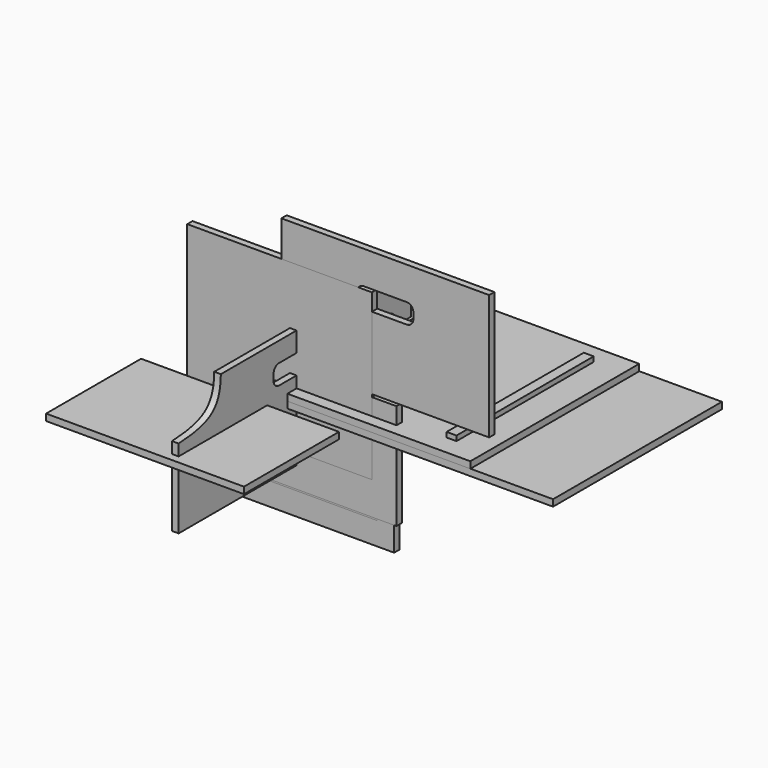
from build123d import *

# Parameters (mm, degrees)
F0_W      = 558.8
F0_H      = 406.4
F0_W_2    = 457.2
F0_H_2    = 19.05
F0_W_3    = 19.05
F0_H_3    = 241.3
F1_DEPTH  = 12.7
F2_DEPTH  = 22.225
F3_DEPTH  = 22.225
F4_DEPTH  = 22.225
F5_W      = 457.2
F5_H      = 406.4
F5_W_2    = 19.05
F5_H_2    = 330.2
F6_DEPTH  = 12.7
F7_DEPTH  = 22.225
F8_DEPTH  = 22.225
F9_W      = 406.4
F9_H      = 165.1
F10_DEPTH = 12.7
F12_DEPTH = 12.7
F13_W     = 381
F13_H     = 228.6
F14_DEPTH = 12.7
F15_W     = 400.05
F15_H     = 241.3
F16_DEPTH = 12.7
F17_W     = 317.5
F17_H     = 203.2
F18_DEPTH = 12.7
F19_W     = 381
F19_H     = 203.2
F20_DEPTH = 12.7
F21_W     = 355.6
F21_H     = 317.5
F22_DEPTH = 12.7


with BuildPart() as f1:
    # F0 (on Top) → F1 (new body)
    with BuildSketch(Plane.XY):
        with Locations((244.6383737266, 168.6325731099)):
            Rectangle(F0_W, F0_H)
        with Locations((206.5383737266, 0.3575731099)):
            Rectangle(F0_W_2, F0_H_2, mode=Mode.SUBTRACT)
        with Locations((206.5383737266, 336.9075731099)):
            Rectangle(F0_W_2, F0_H_2, mode=Mode.SUBTRACT)
        with Locations((489.1133737266, 168.6325731099)):
            Rectangle(F0_W_3, F0_H_3, mode=Mode.SUBTRACT)
    extrude(amount=-F1_DEPTH)

    # F0 (on Top) → F2 (join)
    with BuildSketch(Plane.XY):
        with Locations((206.5383737266, 336.9075731099)):
            Rectangle(F0_W_2, F0_H_2)
    extrude(amount=-F2_DEPTH)

    # F0 (on Top) → F3 (join)
    with BuildSketch(Plane.XY):
        with Locations((489.1133737266, 168.6325731099)):
            Rectangle(F0_W_3, F0_H_3)
    extrude(amount=-F3_DEPTH)

    # F0 (on Top) → F4 (join)
    with BuildSketch(Plane.XY):
        with Locations((206.5383737266, 0.3575731099)):
            Rectangle(F0_W_2, F0_H_2)
    extrude(amount=-F4_DEPTH)


with BuildPart() as f6:
    # F5 (on Top) → F6 (new body)
    with BuildSketch(Plane.XY):
        with Locations((136.398, 168.3692485094)):
            Rectangle(F5_W, F5_H)
        with Locations((9.525, 168.3692485094)):
            Rectangle(F5_W_2, F5_H_2, mode=Mode.SUBTRACT)
        with Locations((298.323, 168.3692485094)):
            Rectangle(F5_W_2, F5_H_2, mode=Mode.SUBTRACT)
    extrude(amount=F6_DEPTH)

    # F5 (on Top) → F7 (join)
    with BuildSketch(Plane.XY):
        with Locations((9.525, 168.3692485094)):
            Rectangle(F5_W_2, F5_H_2)
    extrude(amount=F7_DEPTH)

    # F5 (on Top) → F8 (join)
    with BuildSketch(Plane.XY):
        with Locations((298.323, 168.3692485094)):
            Rectangle(F5_W_2, F5_H_2)
    extrude(amount=F8_DEPTH)


with BuildPart() as f10:
    # F9 (on Front) → F10 (new body)
    with BuildSketch(Plane.XZ):
        with Locations((-2.5245882571, -122.1894112668)):
            Rectangle(F9_W, F9_H)
    extrude(amount=F10_DEPTH)


with BuildPart() as f12:
    # F11 (on Right) → F12 (new body)
    with BuildSketch(Plane.YZ):
        with BuildLine():
            Line((-106.0334625381, 110.8109265052), (-194.9334625381, 110.8109265052))
            add(Edge.make_bspline(
                [(-296.5334625381, 34.6109265052), (-215.7922492521, 38.1965605335), (-196.2180797117, 57.5377674894), (-194.9334625381, 110.8109265052)],
                knots=[0, 0, 0, 0, 127, 127, 127, 127], degree=3))
            Line((-296.5334625381, 34.6109265052), (-296.5334625381, -117.7890734948))
            Line((-296.5334625381, -117.7890734948), (-283.8334625381, -117.7890734948))
            Line((-283.8334625381, -117.7890734948), (173.3665374619, -117.7890734948))
            Line((173.3665374619, -117.7890734948), (217.8165374619, -117.7890734948))
            Line((217.8165374619, -117.7890734948), (236.8665374619, -117.7890734948))
            Line((236.8665374619, -117.7890734948), (262.2665374619, -117.7890734948))
            Line((262.2665374619, -117.7890734948), (262.2665374619, 110.8109265052))
            Line((262.2665374619, 110.8109265052), (205.1165374619, 110.8109265052))
            Line((205.1165374619, 110.8109265052), (186.0665374619, 110.8109265052))
            Line((186.0665374619, 110.8109265052), (-86.9834625381, 110.8109265052))
            Line((-86.9834625381, 110.8109265052), (-106.0334625381, 110.8109265052))
        make_face()
        with BuildLine():
            ThreePointArc((-67.9334625381, 60.0109265052), (-64.2137186591, 68.9911826263), (-55.2334625381, 72.7109265052))
            Line((-55.2334625381, 72.7109265052), (20.9665374619, 72.7109265052))
            ThreePointArc((20.9665374619, 72.7109265052), (29.946793583, 68.9911826263), (33.6665374619, 60.0109265052))
            Line((33.6665374619, 60.0109265052), (33.6665374619, 47.3109265052))
            ThreePointArc((33.6665374619, 47.3109265052), (29.946793583, 38.3306703841), (20.9665374619, 34.6109265052))
            Line((20.9665374619, 34.6109265052), (-55.2334625381, 34.6109265052))
            ThreePointArc((-55.2334625381, 34.6109265052), (-64.2137186591, 38.3306703841), (-67.9334625381, 47.3109265052))
            Line((-67.9334625381, 47.3109265052), (-67.9334625381, 60.0109265052))
        make_face(mode=Mode.SUBTRACT)
        with BuildLine():
            ThreePointArc((186.0665374619, 34.6109265052), (189.7862813409, 43.5911826263), (198.7665374619, 47.3109265052))
            Line((198.7665374619, 47.3109265052), (211.4665374619, 47.3109265052))
            ThreePointArc((211.4665374619, 47.3109265052), (220.446793583, 43.5911826263), (224.1665374619, 34.6109265052))
            Line((224.1665374619, 34.6109265052), (224.1665374619, -41.5890734948))
            ThreePointArc((224.1665374619, -41.5890734948), (220.446793583, -50.5693296159), (211.4665374619, -54.2890734948))
            Line((211.4665374619, -54.2890734948), (198.7665374619, -54.2890734948))
            ThreePointArc((198.7665374619, -54.2890734948), (189.7862813409, -50.5693296159), (186.0665374619, -41.5890734948))
            Line((186.0665374619, -41.5890734948), (186.0665374619, 34.6109265052))
        make_face(mode=Mode.SUBTRACT)
    extrude(amount=F12_DEPTH)


with BuildPart() as f14:
    # F13 (on Top) → F14 (new body)
    with BuildSketch(Plane.XY):
        with Locations((-39.6020258009, -197.6545680389)):
            Rectangle(F13_W, F13_H)
    extrude(amount=F14_DEPTH)


with BuildPart() as f16:
    # F15 (on Front) → F16 (new body)
    with BuildSketch(Plane.XZ):
        with Locations((183.5180822253, 170.7687626004)):
            Rectangle(F15_W, F15_H)
        with BuildLine():
            ThreePointArc((129.5430822253, 215.2187626004), (133.2628261043, 224.1990187215), (142.2430822253, 227.9187626004))
            Line((142.2430822253, 227.9187626004), (224.7930822253, 227.9187626004))
            ThreePointArc((224.7930822253, 227.9187626004), (233.7733383464, 224.1990187215), (237.4930822253, 215.2187626004))
            Line((237.4930822253, 215.2187626004), (237.4930822253, 202.5187626004))
            ThreePointArc((237.4930822253, 202.5187626004), (233.7733383464, 193.5385064794), (224.7930822253, 189.8187626004))
            Line((224.7930822253, 189.8187626004), (142.2430822253, 189.8187626004))
            ThreePointArc((142.2430822253, 189.8187626004), (133.2628261043, 193.5385064794), (129.5430822253, 202.5187626004))
            Line((129.5430822253, 202.5187626004), (129.5430822253, 215.2187626004))
        make_face(mode=Mode.SUBTRACT)
    extrude(amount=F16_DEPTH)


with BuildPart() as f18:
    # F17 (on Front) → F18 (new body)
    with BuildSketch(Plane.XZ):
        with Locations((8.9374314994, -59.3209858673)):
            Rectangle(F17_W, F17_H)
    extrude(amount=F18_DEPTH)


with BuildPart() as f20:
    # F19 (on Front) → F20 (new body)
    with BuildSketch(Plane.XZ):
        with Locations((14.6888829768, -56.5550823708)):
            Rectangle(F19_W, F19_H)
    extrude(amount=F20_DEPTH)


with BuildPart() as f22:
    # F21 (on Front) → F22 (new body)
    with BuildSketch(Plane.XZ):
        with Locations((-19.9289359152, 63.8950824002)):
            Rectangle(F21_W, F21_H)
    extrude(amount=F22_DEPTH)


solid = Compound([f1.part, f6.part, f10.part, f12.part, f14.part, f16.part, f18.part, f20.part, f22.part])
